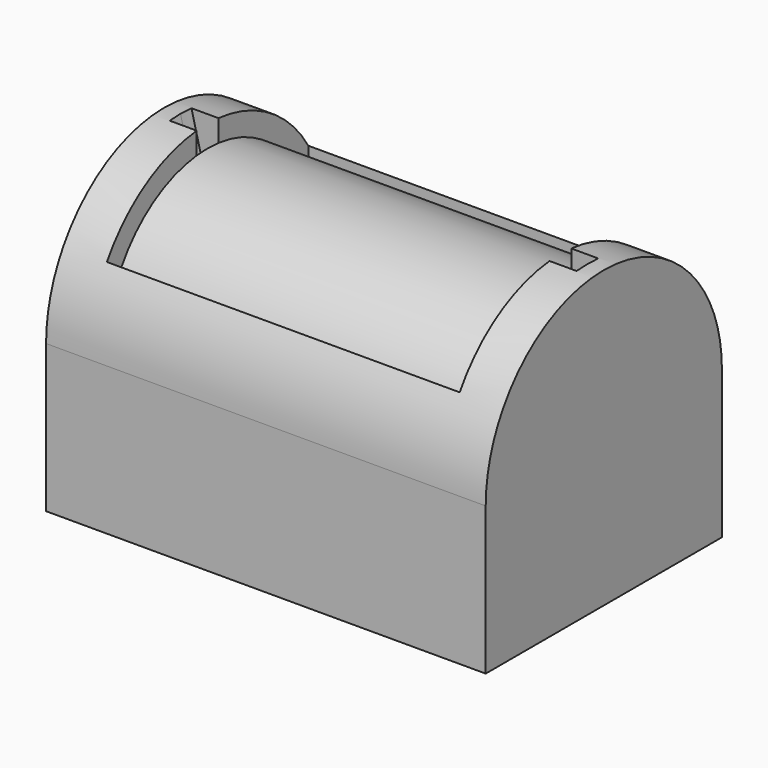
from build123d import *

# Parameters (mm, degrees)
F0_W          = 16.25
F0_H          = 5.8
F3_DEPTH      = 2
F3_DEPTH_BACK = 18.25
F4_DEPTH      = 16.25
F6_DEPTH      = 0.625


with BuildPart() as f1:
    # F0 (on Front) → F1 (revolve)
    with BuildSketch(Plane.XZ):
        with Locations((0, 2.9)):
            Rectangle(F0_W, F0_H)
    revolve(axis=Axis((0, 0, 0), (1, 0, 0)))


with BuildPart() as f3:
    # F2 (on face) → F3 (new body, two sides)
    with BuildSketch(Plane(origin=(-8.125, 0, 0), x_dir=(0, -1, 0), z_dir=(-1, 0, 0))) as f3_sk:
        with BuildLine():
            Line((-3.5, -6.8), (3.5, -6.8))
            Line((3.5, -6.8), (3.5, -4.6249324319))
            ThreePointArc((3.5, -4.6249324319), (0, -5.8), (-3.5, -4.6249324319))
            Line((-3.5, -4.6249324319), (-3.5, -6.8))
        make_face()
        with BuildLine():
            Line((3.5, -6.8), (6.8, -6.8))
            Line((6.8, -6.8), (6.8, 0))
            ThreePointArc((6.8, 0), (6.5452272688, 1.8439088915), (5.8, 3.5496478699))
            Line((5.8, 3.5496478699), (5.8, 0))
            ThreePointArc((5.8, 0), (5.193264869, -2.582634314), (3.5, -4.6249324319))
            Line((3.5, -4.6249324319), (3.5, -6.8))
        make_face()
        with BuildLine():
            Line((-6.8, -6.8), (-3.5, -6.8))
            Line((-3.5, -6.8), (-3.5, -4.6249324319))
            ThreePointArc((-3.5, -4.6249324319), (-5.193264869, -2.582634314), (-5.8, 0))
            Line((-5.8, 0), (-5.8, 3.5496478699))
            ThreePointArc((-5.8, 3.5496478699), (-6.5452272688, 1.8439088915), (-6.8, 0))
            Line((-6.8, 0), (-6.8, -6.8))
        make_face()
        with BuildLine():
            Line((5.8, 0), (5.8, 3.5496478699))
            ThreePointArc((5.8, 3.5496478699), (3.3243341229, 5.9320150572), (4.08e-08, 6.8))
            ThreePointArc((4.08e-08, 6.8), (-3.3243340873, 5.9320150772), (-5.8, 3.5496478699))
            Line((-5.8, 3.5496478699), (-5.8, 0))
            ThreePointArc((-5.8, 0), (0, 5.8), (5.8, 0))
        make_face()
        with BuildLine():
            ThreePointArc((-3.5, -4.6249324319), (0, -5.8), (3.5, -4.6249324319))
            ThreePointArc((3.5, -4.6249324319), (5.193264869, -2.582634314), (5.8, 0))
            ThreePointArc((5.8, 0), (0, 5.8), (-5.8, 0))
            ThreePointArc((-5.8, 0), (-5.193264869, -2.582634314), (-3.5, -4.6249324319))
        make_face()
    extrude(amount=F3_DEPTH)
    extrude(f3_sk.sketch, amount=-F3_DEPTH_BACK)

    # F2 (on face) → F4 (cut, through all)
    with BuildSketch(Plane(origin=(-8.125, 0, 0), x_dir=(0, -1, 0), z_dir=(-1, 0, 0))):
        with BuildLine():
            ThreePointArc((-3.5, -4.6249324319), (0, -5.8), (3.5, -4.6249324319))
            ThreePointArc((3.5, -4.6249324319), (5.193264869, -2.582634314), (5.8, 0))
            ThreePointArc((5.8, 0), (0, 5.8), (-5.8, 0))
            ThreePointArc((-5.8, 0), (-5.193264869, -2.582634314), (-3.5, -4.6249324319))
        make_face()
        with BuildLine():
            Line((5.8, 0), (5.8, 3.5496478699))
            ThreePointArc((5.8, 3.5496478699), (3.3243341229, 5.9320150572), (4.08e-08, 6.8))
            ThreePointArc((4.08e-08, 6.8), (-3.3243340873, 5.9320150772), (-5.8, 3.5496478699))
            Line((-5.8, 3.5496478699), (-5.8, 0))
            ThreePointArc((-5.8, 0), (0, 5.8), (5.8, 0))
        make_face()
        with BuildLine():
            Line((-3.5, -6.8), (3.5, -6.8))
            Line((3.5, -6.8), (3.5, -4.6249324319))
            ThreePointArc((3.5, -4.6249324319), (0, -5.8), (-3.5, -4.6249324319))
            Line((-3.5, -4.6249324319), (-3.5, -6.8))
        make_face()
    extrude(amount=-F4_DEPTH, mode=Mode.SUBTRACT)

    # F5 (on Front) → F6 (cut, symmetric)
    with BuildSketch(Plane.XZ):
        with BuildLine():
            Line((-9.375, -6.8), (-8.125, -6.8))
            Line((-8.125, -6.8), (-8.125, -4.6249324319))
            Line((-8.125, -4.6249324319), (-8.125, 0))
            add(Edge.make_bspline(
                [(-8.125, 0), (-8.125, -2.7403182344), (-8.4223272721, -2.7403182344), (-9.375, -6.8)],
                knots=[0, 0, 0, 0, 6.9139352036, 6.9139352036, 6.9139352036, 6.9139352036], degree=3))
        make_face()
        Polygon((-8.125, -4.6249324319), (-8.125, -6.8), (8.125, -6.8), (8.125, -4.6249324319), (8.125, 0), (8.125, 3.5496478699), (8.125, 6.8), (-8.125, 6.8), (-8.125, 3.5496478699), (-8.125, 0), align=None)
        with BuildLine():
            Line((8.125, -4.6249324319), (8.125, -6.8))
            Line((8.125, -6.8), (9.375, -6.8))
            add(Edge.make_bspline(
                [(8.125, 0), (8.125, -2.7403182344), (8.4223272721, -2.7403182344), (9.375, -6.8)],
                knots=[0, 0, 0, 0, 6.9139352036, 6.9139352036, 6.9139352036, 6.9139352036], degree=3))
            Line((8.125, 0), (8.125, -4.6249324319))
        make_face()
        with BuildLine():
            add(Edge.make_bspline(
                [(-8.125, 0), (-8.125, 2.7403182344), (-8.4223272721, 2.7403182344), (-9.375, 6.8)],
                knots=[0, 0, 0, 0, 6.9139352036, 6.9139352036, 6.9139352036, 6.9139352036], degree=3))
            Line((-8.125, 0), (-8.125, 3.5496478699))
            Line((-8.125, 3.5496478699), (-8.125, 6.8))
            Line((-8.125, 6.8), (-9.375, 6.8))
        make_face()
        with BuildLine():
            Line((8.125, 3.5496478699), (8.125, 0))
            add(Edge.make_bspline(
                [(8.125, 0), (8.125, 2.7403182344), (8.4223272721, 2.7403182344), (9.375, 6.8)],
                knots=[0, 0, 0, 0, 6.9139352036, 6.9139352036, 6.9139352036, 6.9139352036], degree=3))
            Line((9.375, 6.8), (8.125, 6.8))
            Line((8.125, 6.8), (8.125, 3.5496478699))
        make_face()
    extrude(amount=F6_DEPTH, both=True, mode=Mode.SUBTRACT)


solid = Compound([f1.part, f3.part])
